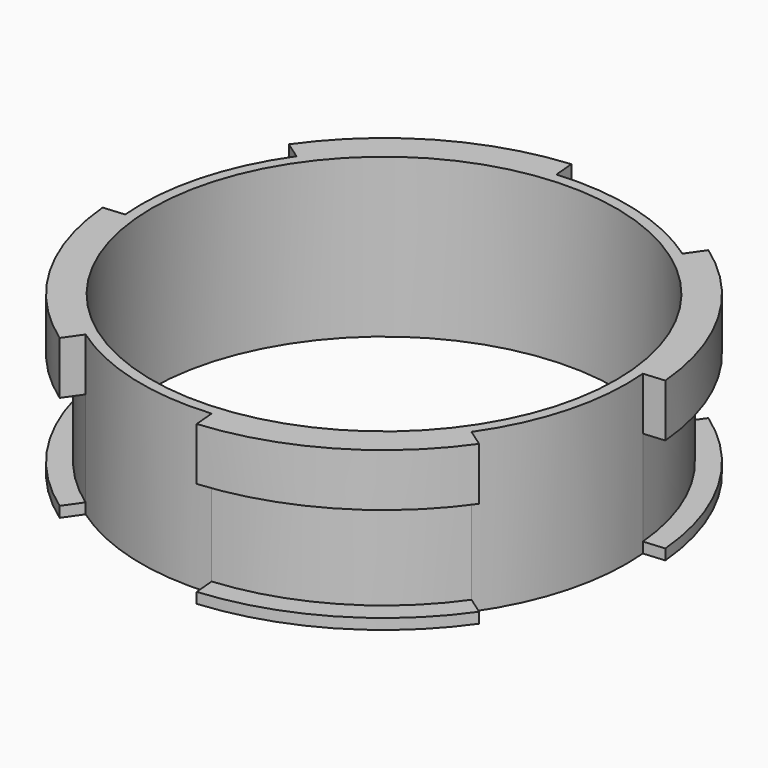
from build123d import *

# Parameters (mm, degrees)
F0_R            = 25
F0_R_2          = 22
F1_DEPTH        = 15
F3_DEPTH        = 15
F3_COPIES_COUNT = 4
F5_R            = 38.565863123
F5_R_2          = 23
F6_DEPTH        = 2.5
F7_R            = 30.9780307995
F7_R_2          = 23
F8_DEPTH        = 4


# Not quite as in the source:
# - a pattern or mirror of a feature is missing from the dataset's text; its kind, count and spacing are read off the source's solid


with BuildPart() as f1:
    # F0 (on Top) → F1 (new body)
    with BuildSketch(Plane.XY):
        Circle(F0_R)
        Circle(F0_R_2, mode=Mode.SUBTRACT)
    extrude(amount=F1_DEPTH)

    # F2 (on Top) → F3 (cut, through all)
    with BuildSketch(Plane.XY):
        with BuildLine():
            Line((13.1922580361, 18.8404970186), (14.3394109088, 20.4788011072))
            ThreePointArc((14.3394109088, 20.4788011072), (6.4704761276, 24.1481456572), (-2.1788935687, 24.9048674523))
            Line((-2.1788935687, 24.9048674523), (-2.0045820832, 22.9124780561))
            ThreePointArc((-2.0045820832, 22.9124780561), (5.9528380374, 22.2162940046), (13.1922580361, 18.8404970186))
        make_face()
    f3 = extrude(amount=F3_DEPTH, mode=Mode.SUBTRACT)

    # F3_copies: F3 ×4 about axis
    f3_copies_axis = Axis((0, 0, 0), (0, 0, 1))
    for i in range(1, F3_COPIES_COUNT):
        add(f3.rotate(f3_copies_axis, i * 360 / F3_COPIES_COUNT), mode=Mode.SUBTRACT)

    # F5 (on offset) → F6 (cut, symmetric)
    with BuildSketch(Plane.XY.offset(7.5)):
        Circle(F5_R)
        Circle(F5_R_2, mode=Mode.SUBTRACT)
    extrude(amount=F6_DEPTH, both=True, mode=Mode.SUBTRACT)

    # F7 (on face) → F8 (cut)
    with BuildSketch(Plane.XY.offset(5)):
        Circle(F7_R)
        Circle(F7_R_2, mode=Mode.SUBTRACT)
    extrude(amount=-F8_DEPTH, mode=Mode.SUBTRACT)


solid = f1.part
